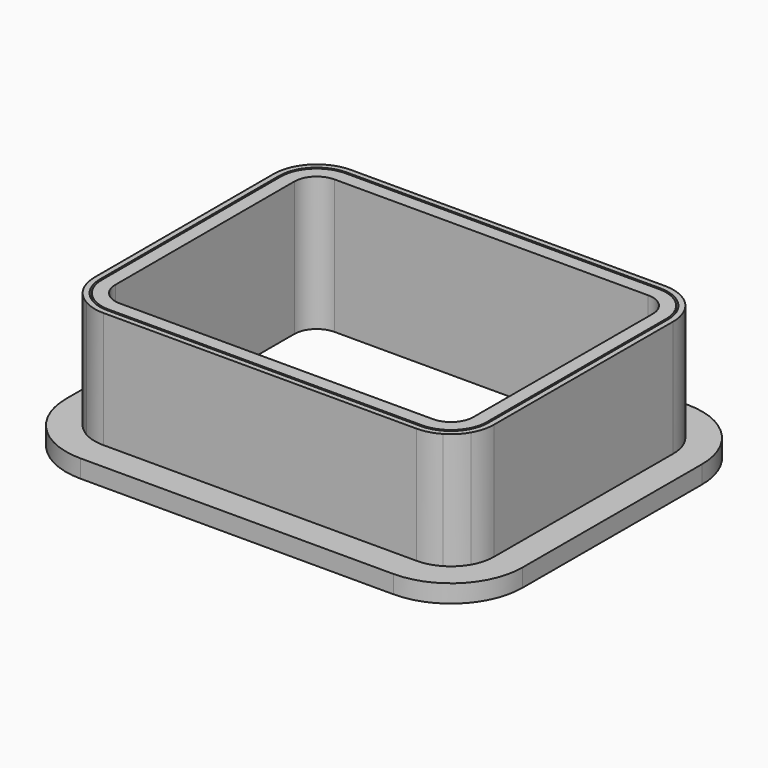
from build123d import *

# Parameters (mm, degrees)
F1_DEPTH = 30
F2_DEPTH = 30
F4_DEPTH = 4


# Not quite as in the source:
# - a feature of the source that left no trace in its solid (it failed there, or was rolled back) is left out


with BuildPart() as f1:
    # F0 (on Top) → F1 (new body)
    with BuildSketch(Plane.XY):
        with BuildLine():
            Line((34.9916597222, 33), (-35.1, 33))
            ThreePointArc((-35.1, 33), (-40.7568542495, 30.6568542495), (-43.1, 25))
            Line((-43.1, 25), (-43.1, -25))
            ThreePointArc((-43.1, -25), (-40.7568542495, -30.6568542495), (-35.1, -33))
            Line((-35.1, -33), (34.9083263889, -33))
            ThreePointArc((34.9083263889, -33), (40.5604646339, -30.6615663256), (42.9083152778, -25.0133333148))
            Line((42.9083152778, -25.0133333148), (42.9916486111, 24.9866666852))
            ThreePointArc((42.9916486111, 24.9866666852), (40.6532260478, 30.652138245), (34.9916597222, 33))
        make_face()
        with BuildLine():
            Line((34.9083263889, -30), (-35.1, -30))
            ThreePointArc((-35.1, -30), (-38.6355339059, -28.5355339059), (-40.1, -25))
            Line((-40.1, -25), (-40.1, 25))
            ThreePointArc((-40.1, 25), (-38.6355339059, 28.5355339059), (-35.1, 30))
            Line((-35.1, 30), (34.9916597222, 30))
            ThreePointArc((34.9916597222, 30), (38.5301386757, 28.5325864031), (39.9916527778, 24.9916666782))
            Line((39.9916527778, 24.9916666782), (39.9083194445, -25.0083333218))
            ThreePointArc((39.9083194445, -25.0083333218), (38.440912792, -28.5384789535), (34.9083263889, -30))
        make_face(mode=Mode.SUBTRACT)
    extrude(amount=F1_DEPTH)


with BuildPart() as f2:
    # F0 (on Top) → F2 (new body)
    with BuildSketch(Plane.XY):
        with BuildLine():
            ThreePointArc((-43.4353358825, 29.7625807841), (-41.1644660941, 31.0644660941), (-39.8625807841, 33.3353358825))
            ThreePointArc((-39.8625807841, 33.3353358825), (-41.8882250994, 31.7882250994), (-43.4353358825, 29.7625807841))
        make_face()
        with BuildLine():
            ThreePointArc((-39.8625807841, -33.3353358825), (-41.1644660941, -31.0644660941), (-43.4353358825, -29.7625807841))
            ThreePointArc((-43.4353358825, -29.7625807841), (-41.8882250994, -31.7882250994), (-39.8625807841, -33.3353358825))
        make_face()
        with BuildLine():
            ThreePointArc((43.3269979462, 29.7625766863), (41.7798801076, 31.7882298134), (39.7542248316, 33.3353448386))
            ThreePointArc((39.7542248316, 33.3353448386), (41.0561149382, 31.0644636388), (43.3269979462, 29.7625766863))
        make_face()
        with BuildLine():
            ThreePointArc((39.7695232115, -33.2782102807), (41.7258186338, -31.7588312222), (43.228235626, -29.7894791247))
            ThreePointArc((43.228235626, -29.7894791247), (41.040869178, -31.0797754051), (39.7695232115, -33.2782102807))
        make_face()
        with BuildLine():
            Line((34.9916597222, 34.6), (-35.1, 34.6))
            ThreePointArc((-35.1, 34.6), (-37.5638156919, 34.2784488055), (-39.8625807841, 33.3353358825))
            ThreePointArc((-39.8625807841, 33.3353358825), (-41.1644660941, 31.0644660941), (-43.4353358825, 29.7625807841))
            ThreePointArc((-43.4353358825, 29.7625807841), (-44.3784488055, 27.4638156919), (-44.7, 25))
            Line((-44.7, 25), (-44.7, -25))
            ThreePointArc((-44.7, -25), (-44.3784488055, -27.4638156919), (-43.4353358825, -29.7625807841))
            ThreePointArc((-43.4353358825, -29.7625807841), (-41.1644660941, -31.0644660941), (-39.8625807841, -33.3353358825))
            ThreePointArc((-39.8625807841, -33.3353358825), (-37.5638156919, -34.2784488055), (-35.1, -34.6))
            Line((-35.1, -34.6), (34.9083263889, -34.6))
            ThreePointArc((34.9083263889, -34.6), (37.4271734769, -34.2636606883), (39.7695232115, -33.2782102807))
            ThreePointArc((39.7695232115, -33.2782102807), (41.040869178, -31.0797754051), (43.228235626, -29.7894791247))
            ThreePointArc((43.228235626, -29.7894791247), (44.1807151368, -27.4865250667), (44.5083130556, -25.0159999778))
            Line((44.5083130556, -25.0159999778), (44.5916463889, 24.9840000222))
            ThreePointArc((44.5916463889, 24.9840000222), (44.2721590874, 27.4560805226), (43.3269979462, 29.7625766863))
            ThreePointArc((43.3269979462, 29.7625766863), (41.0561149382, 31.0644636388), (39.7542248316, 33.3353448386))
            ThreePointArc((39.7542248316, 33.3353448386), (37.45546669, 34.2784511221), (34.9916597222, 34.6))
        make_face()
        with BuildLine():
            ThreePointArc((-43.5, 25), (-41.039696962, 30.939696962), (-35.1, 33.4))
            Line((-35.1, 33.4), (34.9916597222, 33.4))
            ThreePointArc((34.9916597222, 33.4), (40.9363043641, 30.9347451573), (43.3916480556, 24.9860000194))
            Line((43.3916480556, 24.9860000194), (43.3083147223, -25.0139999806))
            ThreePointArc((43.3083147223, -25.0139999806), (40.8430715462, -30.9446446419), (34.9083263889, -33.4))
            Line((34.9083263889, -33.4), (-35.1, -33.4))
            ThreePointArc((-35.1, -33.4), (-41.039696962, -30.939696962), (-43.5, -25))
            Line((-43.5, -25), (-43.5, 25))
        make_face(mode=Mode.SUBTRACT)
    extrude(amount=F2_DEPTH)

    # F3 (on face) → F4 (join)
    with BuildSketch(Plane(origin=(0, 0, 0), x_dir=(1, 0, 0), z_dir=(0, 0, -1))):
        with BuildLine():
            ThreePointArc((-35.1, 41), (-46.413708499, 36.313708499), (-51.1, 25))
            Line((-51.1, 25), (-51.1, -25))
            ThreePointArc((-51.1, -25), (-46.413708499, -36.313708499), (-35.1, -41))
            Line((-35.1, -41), (34.9916597222, -41))
            ThreePointArc((34.9916597222, -41), (46.3147923734, -36.30427649), (50.9916375001, -24.9733333704))
            Line((50.9916375001, -24.9733333704), (50.9083041667, 25.0266666296))
            ThreePointArc((50.9083041667, 25.0266666296), (46.2126028789, 36.3231326512), (34.9083263889, 41))
            Line((34.9083263889, 41), (-35.1, 41))
        make_face()
        with BuildLine():
            Line((-44.7, -25), (-44.7, 25))
            ThreePointArc((-44.7, 25), (-41.8882250994, 31.7882250994), (-35.1, 34.6))
            Line((-35.1, 34.6), (34.9083263889, 34.6))
            ThreePointArc((34.9083263889, 34.6), (41.6908922829, 31.7938795907), (44.5083130556, 25.0159999778))
            Line((44.5083130556, 25.0159999778), (44.5916463889, -24.9840000222))
            ThreePointArc((44.5916463889, -24.9840000222), (41.785539313, -31.782565894), (34.9916597222, -34.6))
            Line((34.9916597222, -34.6), (-35.1, -34.6))
            ThreePointArc((-35.1, -34.6), (-41.8882250994, -31.7882250994), (-44.7, -25))
        make_face(mode=Mode.SUBTRACT)
    extrude(amount=-F4_DEPTH)


solid = Compound([f1.part, f2.part])
